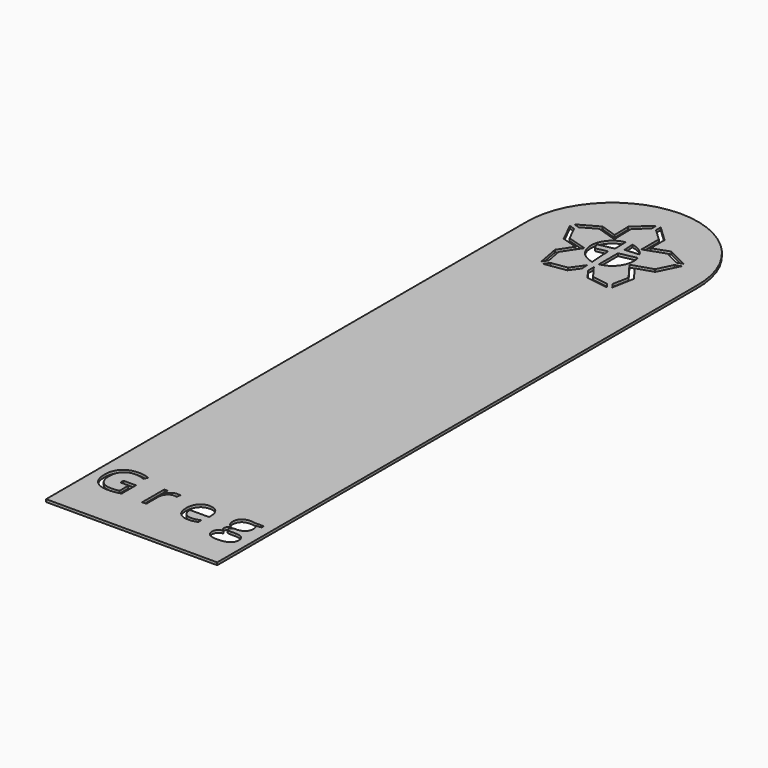
from build123d import *

# Parameters (mm, degrees)
F1_DEPTH     = 0.6
F2_TEXT_SIZE = 12.0661529052
F3_DEPTH     = 25


# Not quite as in the source:
# - Text() gives the source's letters only with a copy of the font that has no kerning and outlines rounded to 1/6400 em; it was checked with that copy


with BuildPart() as f1:
    # F0 (on Top) → F1 (new body)
    with BuildSketch(Plane.XY):
        with BuildLine():
            Line((-6.2929817945, -85.9107411313), (-6.2929817945, 54.0892588687))
            ThreePointArc((-6.2929817945, 54.0892588687), (-26.2881293893, 74.529795656), (-46.2832769841, 54.0892588687))
            Line((-46.2832769841, 54.0892588687), (-46.2832769841, -85.9107411313))
            Line((-46.2832769841, -85.9107411313), (-6.2929817945, -85.9107411313))
        make_face()
        Polygon((-39.1357927602, 58.156282706), (-37.8167754178, 57.7488087208), (-36.0964508727, 54.2858152185), (-31.5504507998, 52.9304291024), (-34.2764975503, 48.8383139018), (-33.5787166392, 45.068726519), (-34.3857806482, 43.9346634595), (-35.333623671, 49.0551490486), (-33.1328767374, 52.3587277484), (-36.798669675, 53.4516808439), align=None, mode=Mode.SUBTRACT)
        Polygon((-33.5710354633, 43.3548442777), (-32.7639714543, 44.4889073372), (-29.0395161137, 45.0546483044), (-26.9457103872, 47.9622273289), (-26.8474352261, 46.3874498879), (-28.4737006293, 44.1291242395), align=None, mode=Mode.SUBTRACT)
        Polygon((-29.5887580141, 64.1036548186), (-29.4783906855, 59.0562246323), (-34.1743482277, 60.578727629), (-37.5216161236, 58.7042567785), (-38.840633466, 59.1117307637), (-34.2816513675, 61.6647618677), (-30.5089220455, 60.4415839222), (-30.598373451, 64.5324659769), (-26.7969193064, 68.043156412), (-26.8055869837, 66.6739480655), align=None, mode=Mode.SUBTRACT)
        with BuildLine():
            Line((-30.0487077198, 54.0772011169), (-27.3612933233, 54.6215970535))
            Line((-27.3612933233, 54.6215970535), (-27.0471519031, 49.5877429627))
            ThreePointArc((-27.0471519031, 49.5877429627), (-31.2879394854, 54.4862181068), (-27.1331783382, 59.4578675177))
            Line((-27.1331783382, 59.4578675177), (-27.0563370558, 56.2451489523))
            Line((-27.0563370558, 56.2451489523), (-30.742992647, 55.4983343463))
            Line((-30.742992647, 55.4983343463), (-30.0487077198, 54.0772011169))
        make_face(mode=Mode.SUBTRACT)
        Polygon((-25.4982272163, 46.435824232), (-25.4982272163, 48.115820707), (-23.2306225225, 45.0546483044), (-19.4864443863, 44.4883009736), (-18.6820422025, 43.3552512513), (-23.7884122058, 44.1276447957), align=None, mode=Mode.SUBTRACT)
        with BuildLine():
            Line((-25.4982272163, 49.5925844435), (-25.4982272163, 55.1695583854))
            Line((-25.4982272163, 55.1695583854), (-21.5027353554, 55.9789346902))
            ThreePointArc((-21.5027353554, 55.9789346902), (-22.0493383686, 51.8778811244), (-25.4982272163, 49.5925844435))
        make_face(mode=Mode.SUBTRACT)
        Polygon((-17.8666377764, 43.9341429699), (-18.6710399602, 45.0671926922), (-17.9616594687, 48.8383139018), (-21.0258079788, 52.9304291024), (-16.2674002349, 54.4754809234), (-14.5643813054, 57.960361879), (-13.2345696342, 58.4039797299), (-15.5551681686, 53.6553480512), (-19.3875651028, 52.4109713225), (-16.8975931641, 49.0856586015), align=None, mode=Mode.SUBTRACT)
        with BuildLine():
            Line((-22.0889890684, 57.2440580909), (-25.3886347637, 56.9700004999))
            Line((-25.3886347637, 56.9700004999), (-25.5972594206, 59.481835507))
            ThreePointArc((-25.5972594206, 59.481835507), (-23.5992705051, 58.7452479332), (-22.0889890684, 57.2440580909))
        make_face(mode=Mode.SUBTRACT)
        Polygon((-13.5510203564, 59.3525886801), (-14.8808320276, 58.9089708292), (-18.3619530872, 60.6872062199), (-23.0988633455, 59.0107087439), (-23.0988633455, 64.1036548186), (-25.8056070202, 66.6676177626), (-25.796939343, 68.0368261091), (-22.0988633455, 64.5338236232), (-22.0988633455, 60.4254140461), (-18.2901023062, 61.7734189524), align=None, mode=Mode.SUBTRACT)
    extrude(amount=F1_DEPTH)

    # F2 (on face) → F3 (cut)
    with BuildSketch(Plane.XY.offset(0.6)):
        with Locations((-44.7832769841, -75.9107411313)):
            Text('G r e g', F2_TEXT_SIZE, font='Open Sans', text_align=(TextAlign.LEFT, TextAlign.BOTTOM))
        with BuildLine():
            add(Edge.make_bspline(
                [(-13.3528340025, -76.0813640748), (-13.7242452716, -76.3990432567), (-13.7242452716, -76.9948095564)],
                knots=[0, 0, 0, 1, 1, 1], degree=2))
            add(Edge.make_bspline(
                [(-13.7242452716, -76.9948095564), (-13.7242452716, -77.5189330732), (-13.2821338878, -77.7904215136)],
                knots=[0, 0, 0, 1, 1, 1], degree=2))
            add(Edge.make_bspline(
                [(-13.2821338878, -77.7904215136), (-12.840022504, -78.061909954), (-12.0161305009, -78.061909954)],
                knots=[0, 0, 0, 1, 1, 1], degree=2))
            add(Edge.make_bspline(
                [(-12.0161305009, -78.061909954), (-10.7850058373, -78.061909954), (-10.1930102104, -77.6933266894)],
                knots=[0, 0, 0, 1, 1, 1], degree=2))
            add(Edge.make_bspline(
                [(-10.1930102104, -77.6933266894), (-9.6010145835, -77.3247434249), (-9.6010145835, -76.6950410702)],
                knots=[0, 0, 0, 1, 1, 1], degree=2))
            add(Edge.make_bspline(
                [(-9.6010145835, -76.6950410702), (-9.6010145835, -76.1709175533), (-9.9243497746, -75.9673012231)],
                knots=[0, 0, 0, 1, 1, 1], degree=2))
            add(Edge.make_bspline(
                [(-9.9243497746, -75.9673012231), (-10.2476849658, -75.7636848928), (-11.1432197517, -75.7636848928)],
                knots=[0, 0, 0, 1, 1, 1], degree=2))
            Line((-11.1432197517, -75.7636848928), (-12.3158989872, -75.7636848928))
            add(Edge.make_bspline(
                [(-12.3158989872, -75.7636848928), (-12.9814227334, -75.7636848928), (-13.3528340025, -76.0813640748)],
                knots=[0, 0, 0, 1, 1, 1], degree=2))
        make_face()
        with BuildLine():
            add(Edge.make_bspline(
                [(-12.8230544765, -70.4196988913), (-13.1944657456, -70.7901674922), (-13.1944657456, -71.5216780121)],
                knots=[0, 0, 0, 1, 1, 1], degree=2))
            add(Edge.make_bspline(
                [(-13.1944657456, -71.5216780121), (-13.1944657456, -72.1985137766), (-12.8117424581, -72.5463583408)],
                knots=[0, 0, 0, 1, 1, 1], degree=2))
            add(Edge.make_bspline(
                [(-12.8117424581, -72.5463583408), (-12.4290191707, -72.894202905), (-11.7446420606, -72.894202905)],
                knots=[0, 0, 0, 1, 1, 1], degree=2))
            add(Edge.make_bspline(
                [(-11.7446420606, -72.894202905), (-10.3136717395, -72.894202905), (-10.3136717395, -71.5028246482)],
                knots=[0, 0, 0, 1, 1, 1], degree=2))
            add(Edge.make_bspline(
                [(-10.3136717395, -71.5028246482), (-10.3136717395, -70.0492302904), (-11.7616100881, -70.0492302904)],
                knots=[0, 0, 0, 1, 1, 1], degree=2))
            add(Edge.make_bspline(
                [(-11.7616100881, -70.0492302904), (-12.4516432074, -70.0492302904), (-12.8230544765, -70.4196988913)],
                knots=[0, 0, 0, 1, 1, 1], degree=2))
        make_face()
        with BuildLine():
            add(Edge.make_bspline(
                [(-20.1240196523, -70.6468819264), (-20.5359656538, -70.1548091283), (-21.3032975652, -70.1548091283)],
                knots=[0, 0, 0, 1, 1, 1], degree=2))
            add(Edge.make_bspline(
                [(-21.3032975652, -70.1548091283), (-22.0800561584, -70.1548091283), (-22.5429062425, -70.6610219494)],
                knots=[0, 0, 0, 1, 1, 1], degree=2))
            add(Edge.make_bspline(
                [(-22.5429062425, -70.6610219494), (-23.0057563266, -71.1672347705), (-23.0887111278, -72.0627695564)],
                knots=[0, 0, 0, 1, 1, 1], degree=2))
            Line((-23.0887111278, -72.0627695564), (-19.7120736508, -72.0627695564))
            add(Edge.make_bspline(
                [(-19.7120736508, -72.0627695564), (-19.7120736508, -71.1389547246), (-20.1240196523, -70.6468819264)],
                knots=[0, 0, 0, 1, 1, 1], degree=2))
        make_face()
    extrude(amount=-F3_DEPTH, mode=Mode.SUBTRACT)


solid = f1.part
